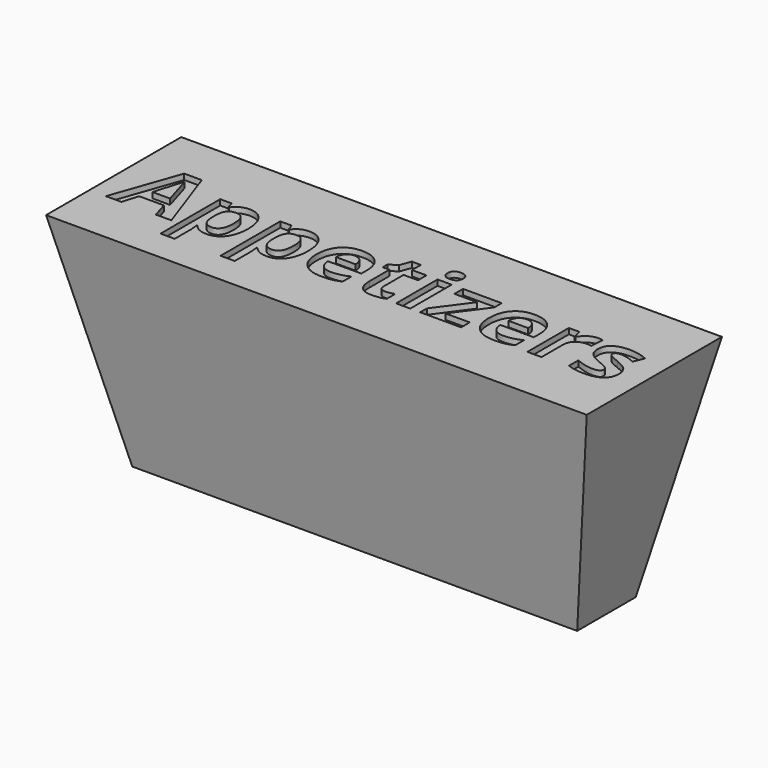
from build123d import *

# Parameters (mm, degrees)
F0_W         = 2438.4
F0_H         = 762
F1_DEPTH     = 1016
F1_TAPER     = 12
F2_TEXT_SIZE = 427.9145949108
F3_DEPTH     = 25.4


# Not quite as in the source:
# - Text() gives the source's letters only with a copy of the font that has no kerning and outlines rounded to 1/6400 em; it was checked with that copy


with BuildPart() as f1:
    # F0 (on Top) → F1 (new body)
    with BuildSketch(Plane.XY):
        Rectangle(F0_W, F0_H)
    extrude(amount=-F1_DEPTH, taper=F1_TAPER)

    # F2 (on face) → F3 (cut)
    with BuildSketch(Plane.XY):
        with Locations((-1144.9535126378, -136.5855039375)):
            Text('Appetizers', F2_TEXT_SIZE, font='Open Sans', font_style=FontStyle.BOLD, text_align=(TextAlign.LEFT, TextAlign.BOTTOM))
    extrude(amount=-F3_DEPTH, mode=Mode.SUBTRACT)


solid = f1.part
